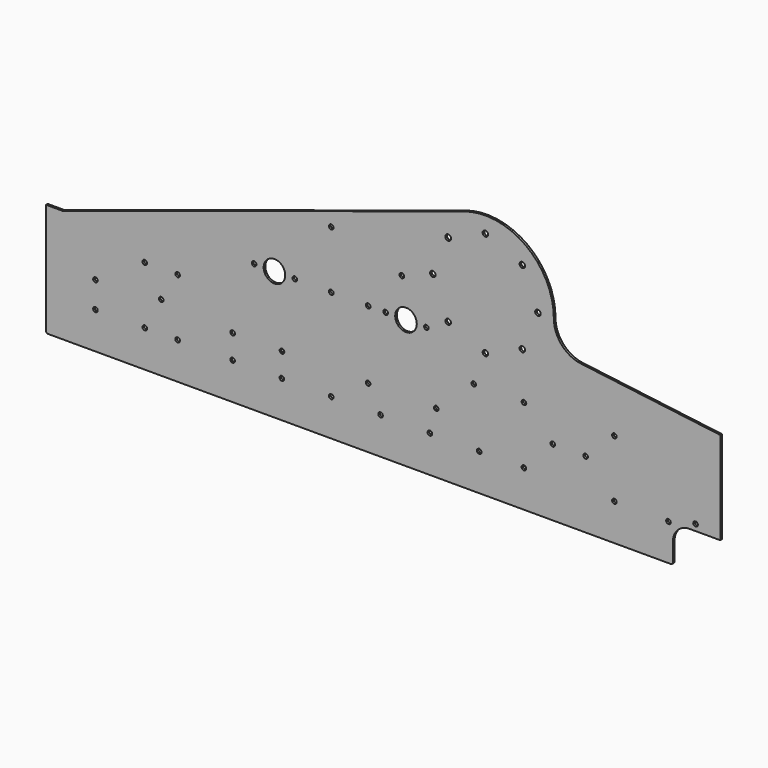
from build123d import *

# Parameters (mm, degrees)
F0_R     = 7.14375
F0_R_2   = 33.3375
F0_R_3   = 8.509
F0_R_4   = 8.89
F1_DEPTH = 6.35


# Not quite as in the source:
# - ends of sketch curves that miss each other by under 0.0002 mm in the source are joined


with BuildPart() as f1:
    # F0 (on Front) → F1 (new body)
    with BuildSketch(Plane.XZ):
        with BuildLine():
            Line((-990.675184, -31.5729874), (-1041.475184, -31.5729874))
            Line((-1041.475184, -31.5729874), (-1041.475184, -374.4729874))
            ThreePointArc((-1041.475184, -374.4729874), (-1039.6153120605, -378.9631154605), (-1035.125184, -380.8229874))
            Line((-1035.125184, -380.8229874), (888.924816, -380.8229874))
            ThreePointArc((888.924816, -380.8229874), (893.4149440605, -378.9631154605), (895.274816, -374.4729874))
            Line((895.274816, -374.4729874), (895.274816, -317.3229874))
            ThreePointArc((895.274816, -317.3229874), (910.1537915157, -281.4019629157), (946.074816, -266.5229874))
            Line((946.074816, -266.5229874), (1041.4752094, -266.5229874))
            Line((1041.4752094, -266.5229874), (1041.4752094, 19.626326))
            Line((1041.4752094, 19.626326), (611.3003013693, 73.7272843556))
            ThreePointArc((611.3003013693, 73.7272843556), (551.322654557, 105.4521002182), (527.3308478102, 168.920007602))
            ThreePointArc((527.3308478102, 168.920007602), (527.3308670888, 168.9390000629), (527.3308558827, 168.9579925234))
            ThreePointArc((527.3308558827, 168.9579925234), (439.9522285654, 340.3269099665), (249.9729787047, 370.4966796024))
            Line((249.9729787047, 370.4966796024), (-990.675184, -31.5729874))
        make_face()
        with Locations((-889.0246634, -266.991084)):
            Circle(F0_R, mode=Mode.SUBTRACT)
        with Locations((-736.6246634, -266.991084)):
            Circle(F0_R, mode=Mode.SUBTRACT)
        with Locations((-635.069342, -266.9311654)):
            Circle(F0_R, mode=Mode.SUBTRACT)
        with Locations((-465.2920082, -266.8996694)):
            Circle(F0_R, mode=Mode.SUBTRACT)
        with Locations((-312.8920082, -266.8996694)):
            Circle(F0_R, mode=Mode.SUBTRACT)
        with Locations((-465.010881, -192.5398994)):
            Circle(F0_R, mode=Mode.SUBTRACT)
        with Locations((-312.610881, -192.5398994)):
            Circle(F0_R, mode=Mode.SUBTRACT)
        with Locations((-160.4920082, -266.8996694)):
            Circle(F0_R, mode=Mode.SUBTRACT)
        with Locations((-8.0920082, -266.8996694)):
            Circle(F0_R, mode=Mode.SUBTRACT)
        with Locations((-46.3986626, -193.1547064)):
            Circle(F0_R, mode=Mode.SUBTRACT)
        with Locations((-888.8878082, -186.200796)):
            Circle(F0_R, mode=Mode.SUBTRACT)
        with Locations((-685.8404368, -173.2472278)):
            Circle(F0_R, mode=Mode.SUBTRACT)
        with Locations((-736.5858268, -89.1617978)):
            Circle(F0_R, mode=Mode.SUBTRACT)
        with Locations((-635.0111506, -89.2015996)):
            Circle(F0_R, mode=Mode.SUBTRACT)
        with Locations((144.3079918, -266.8996694)):
            Circle(F0_R, mode=Mode.SUBTRACT)
        with Locations((163.915471, -193.1547064)):
            Circle(F0_R, mode=Mode.SUBTRACT)
        with Locations((296.7079918, -266.8996694)):
            Circle(F0_R, mode=Mode.SUBTRACT)
        with Locations((434.869844, -266.86002)):
            Circle(F0_R, mode=Mode.SUBTRACT)
        with Locations((714.3297118, -266.927076)):
            Circle(F0_R, mode=Mode.SUBTRACT)
        with Locations((881.4062128, -267.5829294)):
            Circle(F0_R, mode=Mode.SUBTRACT)
        with Locations((965.0764544, -247.1495184)):
            Circle(F0_R, mode=Mode.SUBTRACT)
        with Locations((279.9671566, -89.1229866)):
            Circle(F0_R, mode=Mode.SUBTRACT)
        with Locations((434.915945, -89.109677)):
            Circle(F0_R, mode=Mode.SUBTRACT)
        with Locations((523.8131764, -173.234477)):
            Circle(F0_R, mode=Mode.SUBTRACT)
        with Locations((625.4303722, -173.2491836)):
            Circle(F0_R, mode=Mode.SUBTRACT)
        with Locations((714.2706314, -89.1516632)):
            Circle(F0_R, mode=Mode.SUBTRACT)
        with Locations((-398.852898, 17.0261788)):
            Circle(F0_R, mode=Mode.SUBTRACT)
        with Locations((-335.9403238, 17.0261788)):
            Circle(F0_R_2, mode=Mode.SUBTRACT)
        with Locations((-273.027775, 17.0261788)):
            Circle(F0_R, mode=Mode.SUBTRACT)
        with Locations((-160.4810608, 17.0261788)):
            Circle(F0_R, mode=Mode.SUBTRACT)
        with Locations((-46.3986626, 17.0261788)):
            Circle(F0_R, mode=Mode.SUBTRACT)
        with Locations((-160.4982312, 194.9087288)):
            Circle(F0_R, mode=Mode.SUBTRACT)
        with Locations((7.547102, 17.0261788)):
            Circle(F0_R, mode=Mode.SUBTRACT)
        with Locations((70.4596762, 17.0261788)):
            Circle(F0_R_2, mode=Mode.SUBTRACT)
        with Locations((133.372225, 17.0261788)):
            Circle(F0_R, mode=Mode.SUBTRACT)
        with Locations((200.8515922, 54.1913826)):
            Circle(F0_R_3, mode=Mode.SUBTRACT)
        with Locations((315.8054136, 6.5158112)):
            Circle(F0_R_3, mode=Mode.SUBTRACT)
        with Locations((429.82642, 54.206775)):
            Circle(F0_R_3, mode=Mode.SUBTRACT)
        with Locations((57.5594988, 133.1437774)):
            Circle(F0_R, mode=Mode.SUBTRACT)
        with Locations((153.3248902, 168.9963346)):
            Circle(F0_R_3, mode=Mode.SUBTRACT)
        with Locations((478.0577434, 168.9963346)):
            Circle(F0_R_3, mode=Mode.SUBTRACT)
        with Locations((200.7754176, 283.379291)):
            Circle(F0_R_4, mode=Mode.SUBTRACT)
        with Locations((429.929163, 283.4136826)):
            Circle(F0_R_3, mode=Mode.SUBTRACT)
        with Locations((315.7209586, 331.3233658)):
            Circle(F0_R_3, mode=Mode.SUBTRACT)
    extrude(amount=F1_DEPTH)


solid = f1.part
